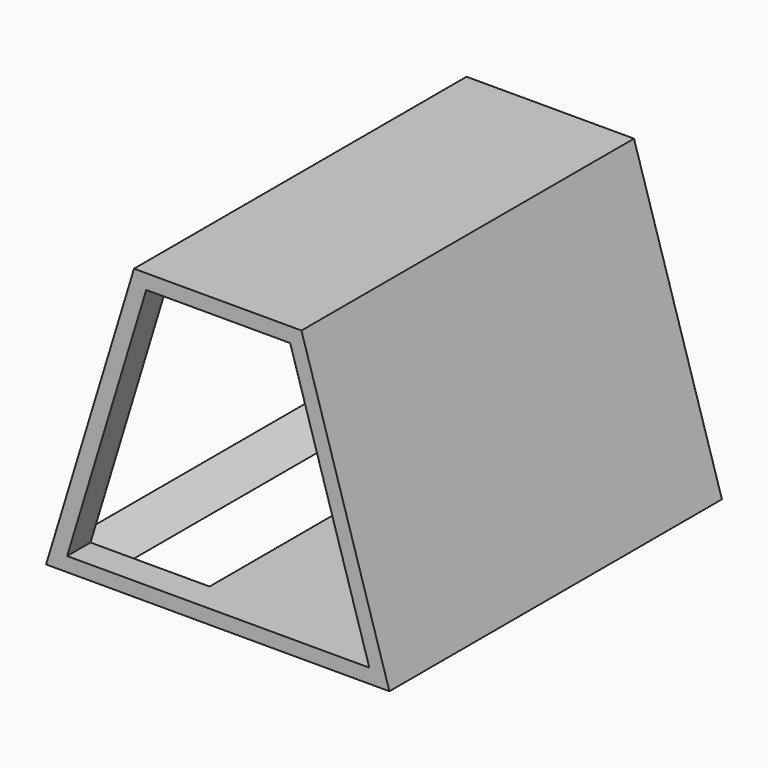
from build123d import *

# Parameters (mm, degrees)
F1_DEPTH = 80
F3_DEPTH = 80
F4_W     = 70.0248382054
F4_H     = 52.043965552
F5_DEPTH = 25


with BuildPart() as f1:
    # F0 (on Front) → F1 (new body)
    with BuildSketch(Plane.XZ):
        Polygon((-16.1164440215, 55.6217506528), (-33.0398865044, 0), (0, 0), (0, 55.6217506528), align=None)
        Polygon((0, 55.6217506528), (0, 0), (33.0398865044, 0), (16.1164440215, 55.6217506528), align=None)
    extrude(amount=F1_DEPTH)

    # F2 (on face) → F3 (cut)
    with BuildSketch(Plane.XZ.offset(80)):
        Polygon((-13.7641547164, 52.7867953574), (-28.990626716, 2.7424246723), (29.1717245215, 2.7424246723), (13.9452525218, 52.7867953574), align=None)
    extrude(amount=-F3_DEPTH, mode=Mode.SUBTRACT)

    # F4 (on face) → F5 (cut)
    with BuildSketch(Plane(origin=(-30.2404161362, 0, 9.200931958), x_dir=(0, -1, 0), z_dir=(-0.9566974319, 0, 0.2910842211))):
        with Locations((39.3633369822, 19.0598971676)):
            Rectangle(F4_W, F4_H)
    extrude(amount=-F5_DEPTH, mode=Mode.SUBTRACT)


solid = f1.part
